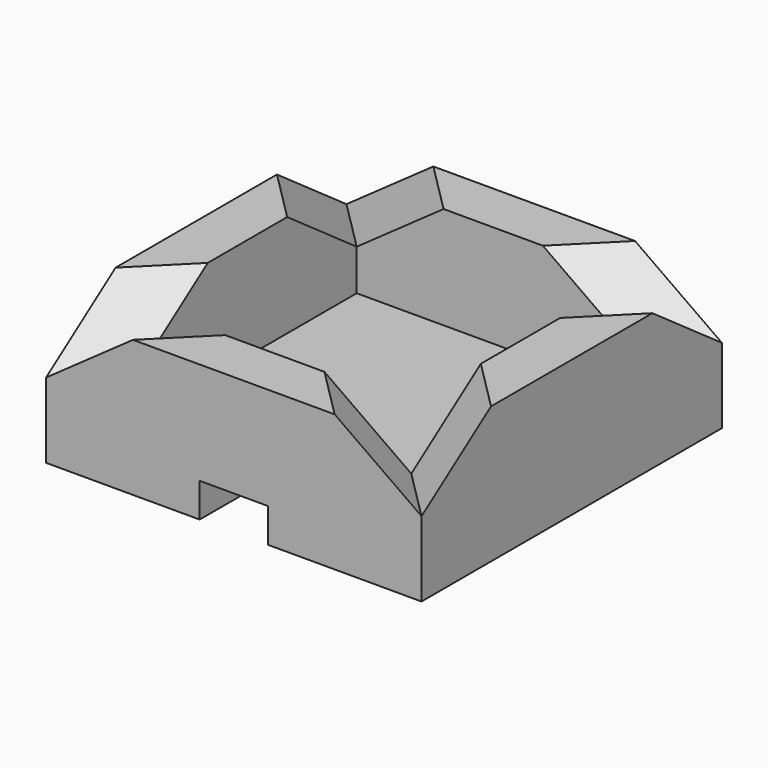
from build123d import *

# Parameters (mm, degrees)
F0_W     = 110
F0_H     = 110
F0_W_2   = 80
F0_H_2   = 80
F1_DEPTH = 40
F0_W_3   = 70
F0_H_3   = 70
F2_DEPTH = 10
F5_DEPTH = 200
F6_W     = 20
F6_H     = 20
F7_DEPTH = 25


# Not quite as in the source:
# - a pattern or mirror of a feature is missing from the dataset's text; its kind, count and spacing are read off the source's solid


with BuildPart() as f1:
    # F0 (on Top) → F1 (new body)
    with BuildSketch(Plane.XY):
        Rectangle(F0_W, F0_H)
        Rectangle(F0_W_2, F0_H_2, mode=Mode.SUBTRACT)
    extrude(amount=F1_DEPTH)

    # F4 (on face) → F5 (cut)
    with BuildSketch(Plane(origin=(55, -55, 0), x_dir=(-0.7071067812, -0.7071067812, 0), z_dir=(-0.7071067812, 0.7071067812, 0))):
        Polygon((-18, 40), (0, 22), (0, 40), align=None)
        Polygon((0, 40), (0, 22), (18, 40), align=None)
    f5 = extrude(amount=F5_DEPTH, mode=Mode.SUBTRACT)

    # F5_copies: F5 across plane
    add(f5.mirror(Plane(origin=(0, 0, 0), x_dir=(0, 0, 1), z_dir=(1, 0, 0))), mode=Mode.SUBTRACT)

    # F6 (on face) → F7 (cut)
    with BuildSketch(Plane.XZ.offset(55)):
        Rectangle(F6_W, F6_H)
    extrude(amount=-F7_DEPTH, mode=Mode.SUBTRACT)


with BuildPart() as f2:
    # F0 (on Top) → F2 (new body)
    with BuildSketch(Plane.XY):
        Rectangle(F0_W_2, F0_H_2)
        Rectangle(F0_W_3, F0_H_3, mode=Mode.SUBTRACT)
        Rectangle(F0_W_3, F0_H_3)
    extrude(amount=F2_DEPTH)


solid = Compound([f1.part, f2.part])
